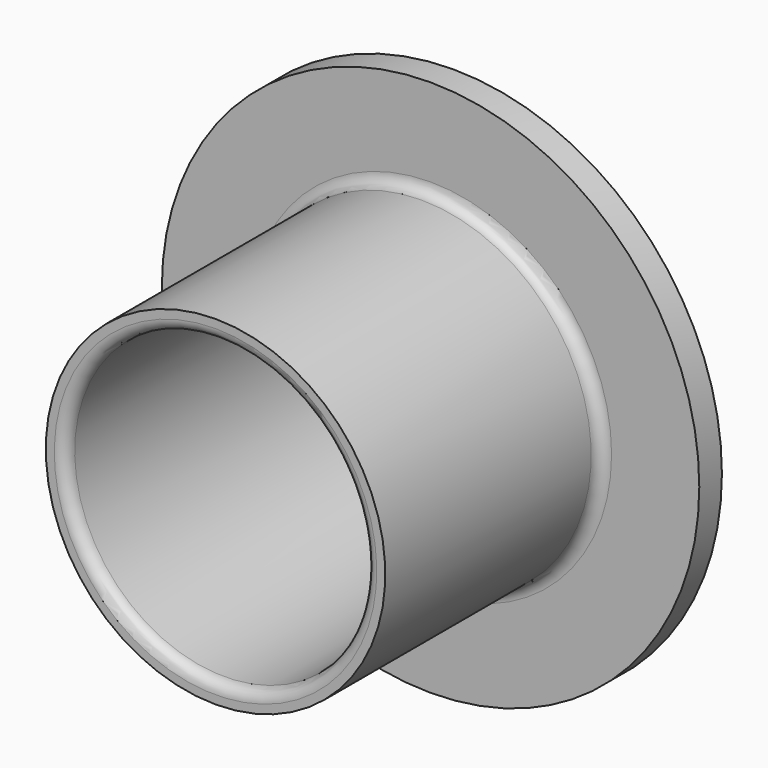
from build123d import *


# Not quite as in the source:
# - a feature of the source that left no trace in its solid (it failed there, or was rolled back) is left out


with BuildPart() as f1:
    # F0 (on Right) → F1 (revolve)
    with BuildSketch(Plane.YZ):
        with BuildLine():
            Line((4.8, 39.2), (0, 39.2))
            Line((0, 39.2), (0, 47.5))
            Line((0, 47.5), (-5, 47.5))
            Line((-5, 47.5), (-5, 32))
            ThreePointArc((-5, 32), (-5.5857864376, 30.5857864376), (-7, 30))
            Line((-7, 30), (-52.5, 30))
            Line((-52.5, 30), (-52.5, 28.5))
            ThreePointArc((-52.5, 28.5), (-51.9142135624, 27.0857864376), (-50.5, 26.5))
            Line((-50.5, 26.5), (0.8, 26.5))
            ThreePointArc((0.8, 26.5), (3.6284271247, 27.6715728753), (4.8, 30.5))
            Line((4.8, 30.5), (4.8, 39.2))
        make_face()
    revolve(axis=Axis((0, -35.2283529937, 0), (0, -1, 0)))


solid = f1.part
